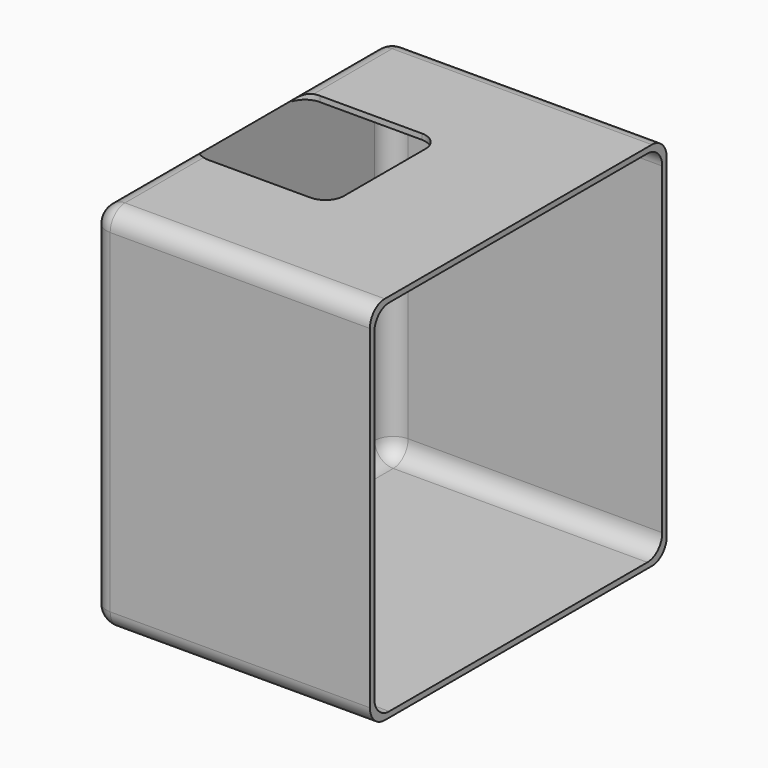
from build123d import *

# Parameters (mm, degrees)
F0_W          = 101.6
F0_H          = 101.6
F0_W_2        = 98.552
F0_H_2        = 98.552
F1_DEPTH      = 76.2
F2_W          = 101.6
F2_H          = 101.6
F3_DEPTH      = 1.524
F4_W          = 38.1
F4_H          = 38.1
F5_DEPTH      = 1.524
F6_R          = 5.08
F7_R          = 5.08
F10_T1_DEPTH  = 93.472
F10_T3_DEPTH  = 88.392
F10_T5_DEPTH  = 74.676
F10_T7_DEPTH  = 69.596
F10_S11_W     = 5.08
F10_S11_H     = 5.08
F10_T12_DEPTH = 5.08
F10_S17_W     = 5.08
F10_S17_H     = 5.08
F10_T18_DEPTH = 5.08
F10_T21_DEPTH = 91.44
F10_T23_DEPTH = 91.44
F10_T26_ANGLE = 90
F10_T28_ANGLE = 90
F10_T30_ANGLE = 90
F10_T32_ANGLE = 90


# Not quite as in the source:
# - a fillet or chamfer that OpenCascade refuses, or shapes differently, is made with other operations: its cross-section is extruded or revolved along the edge and cut away or added
# - a feature of the source that left no trace in its solid (it failed there, or was rolled back) is left out


with BuildPart() as f1:
    # F0 (on Right) → F1 (new body)
    with BuildSketch(Plane.YZ):
        Rectangle(F0_W, F0_H)
        Rectangle(F0_W_2, F0_H_2, mode=Mode.SUBTRACT)
    extrude(amount=F1_DEPTH)

    # F2 (on Right) → F3 (join)
    with BuildSketch(Plane.YZ):
        Rectangle(F2_W, F2_H)
    extrude(amount=F3_DEPTH)

    # F4 (on face) → F5 (cut)
    with BuildSketch(Plane.XY.offset(50.8)):
        with Locations((20.574, 0)):
            Rectangle(F4_W, F4_H)
    extrude(amount=-F5_DEPTH, mode=Mode.SUBTRACT)

    # F6
    f6_edges = [f1.edges().sort_by_distance(p)[0] for p in [
        (39.624, 19.05, 50.038),
        (39.624, -19.05, 50.038),
        (1.524, -19.05, 50.038),
        (1.524, 19.05, 50.038),
    ]]
    fillet(f6_edges, radius=F6_R)

    # F7
    f7_edges = [f1.edges().sort_by_distance(p)[0] for p in [
        (38.1, 50.8, 50.8),
        (38.1, -50.8, 50.8),
        (38.1, -50.8, -50.8),
        (38.1, 50.8, -50.8),
    ]]
    fillet(f7_edges, radius=F7_R)

    # F10: fillet of radius 5.08 on 15 edges, made by hand

    # F10_s2 → F10_t1 (join)
    with BuildSketch(Plane.XY.offset(-44.196)):
        with BuildLine():
            ThreePointArc((1.524, 44.196), (3.0118975516, 47.7881024484), (6.604, 49.276))
            Line((6.604, 49.276), (1.524, 49.276))
            Line((1.524, 49.276), (1.524, 44.196))
        make_face()
        with BuildLine():
            ThreePointArc((1.524, -44.196), (3.0118975516, -47.7881024484), (6.604, -49.276))
            Line((6.604, -49.276), (1.524, -49.276))
            Line((1.524, -49.276), (1.524, -44.196))
        make_face()
    extrude(amount=F10_T1_DEPTH)

    # F10_s4 → F10_t3 (join)
    with BuildSketch(Plane.XZ.offset(-44.196)):
        with BuildLine():
            ThreePointArc((1.524, -44.196), (3.0118975516, -47.7881024484), (6.604, -49.276))
            Line((6.604, -49.276), (1.524, -49.276))
            Line((1.524, -49.276), (1.524, -44.196))
        make_face()
    extrude(amount=F10_T3_DEPTH)

    # F10_s6 → F10_t5 (join)
    with BuildSketch(Plane.YZ.offset(1.524)):
        with BuildLine():
            ThreePointArc((-49.276, 44.196), (-47.7881024484, 47.7881024484), (-44.196, 49.276))
            Line((-44.196, 49.276), (-49.276, 49.276))
            Line((-49.276, 49.276), (-49.276, 44.196))
        make_face()
        with BuildLine():
            ThreePointArc((44.196, 49.276), (47.7881024484, 47.7881024484), (49.276, 44.196))
            Line((49.276, 44.196), (49.276, 49.276))
            Line((49.276, 49.276), (44.196, 49.276))
        make_face()
    extrude(amount=F10_T5_DEPTH)

    # F10_s8 → F10_t7 (join)
    with BuildSketch(Plane.YZ.offset(6.604)):
        with BuildLine():
            ThreePointArc((-49.276, -44.196), (-47.7881024484, -47.7881024484), (-44.196, -49.276))
            Line((-44.196, -49.276), (-49.276, -49.276))
            Line((-49.276, -49.276), (-49.276, -44.196))
        make_face()
        with BuildLine():
            ThreePointArc((49.276, -44.196), (47.7881024484, -47.7881024484), (44.196, -49.276))
            Line((44.196, -49.276), (49.276, -49.276))
            Line((49.276, -49.276), (49.276, -44.196))
        make_face()
    extrude(amount=F10_T7_DEPTH)


with BuildPart() as f10_tool10:
    # F10_s11 → F10_t12 (new body)
    with BuildSketch(Plane.XY.offset(-44.196)):
        with Locations((4.064, 46.736)):
            Rectangle(F10_S11_W, F10_S11_H)
    extrude(amount=-F10_T12_DEPTH)

    # F10_s13 → F10_t14 (revolve, cut)
    with BuildSketch(Plane(origin=(6.604, 44.196, -44.196), x_dir=(0.7071067812, -0.7071067812, 0), z_dir=(0.7071067812, 0.7071067812, 0))):
        with BuildLine():
            ThreePointArc((0, -5.08), (5.08, 0), (0, 5.08))
            Line((0, 5.08), (0, -5.08))
        make_face()
    revolve(axis=Axis((6.604, 44.196, -44.196), (0, 0, -1)), mode=Mode.SUBTRACT)


with BuildPart() as f1_1:
    add(f1.part)

    # F10_t9: union F10_tool10
    add(f10_tool10.part)


with BuildPart() as f10_tool16:
    # F10_s17 → F10_t18 (new body)
    with BuildSketch(Plane.XY.offset(-44.196)):
        with Locations((4.064, -46.736)):
            Rectangle(F10_S17_W, F10_S17_H)
    extrude(amount=-F10_T18_DEPTH)

    # F10_s19 → F10_t20 (revolve, cut)
    with BuildSketch(Plane(origin=(6.604, -44.196, -44.196), x_dir=(0.7071067812, 0.7071067812, 0), z_dir=(-0.7071067812, 0.7071067812, 0))):
        with BuildLine():
            ThreePointArc((0, -5.08), (5.08, 0), (0, 5.08))
            Line((0, 5.08), (0, -5.08))
        make_face()
    revolve(axis=Axis((6.604, -44.196, -44.196), (0, 0, -1)), mode=Mode.SUBTRACT)


with BuildPart() as f1_2:
    add(f1_1.part)

    # F10_t15: union F10_tool16
    add(f10_tool16.part)

    # F10_s22 → F10_t21 (cut)
    with BuildSketch(Plane.XZ.offset(-45.72)):
        with BuildLine():
            ThreePointArc((5.08, 50.8), (1.4878975516, 49.3121024484), (0, 45.72))
            Line((0, 45.72), (0, 50.8))
            Line((0, 50.8), (5.08, 50.8))
        make_face()
        with BuildLine():
            ThreePointArc((5.08, -50.8), (1.4878975516, -49.3121024484), (0, -45.72))
            Line((0, -45.72), (0, -50.8))
            Line((0, -50.8), (5.08, -50.8))
        make_face()
    extrude(amount=F10_T21_DEPTH, mode=Mode.SUBTRACT)

    # F10_s24 → F10_t23 (cut)
    with BuildSketch(Plane.XY.offset(-45.72)):
        with BuildLine():
            ThreePointArc((5.08, 50.8), (1.4878975516, 49.3121024484), (0, 45.72))
            Line((0, 45.72), (0, 50.8))
            Line((0, 50.8), (5.08, 50.8))
        make_face()
        with BuildLine():
            ThreePointArc((5.08, -50.8), (1.4878975516, -49.3121024484), (0, -45.72))
            Line((0, -45.72), (0, -50.8))
            Line((0, -50.8), (5.08, -50.8))
        make_face()
    extrude(amount=F10_T23_DEPTH, mode=Mode.SUBTRACT)

    # F10_s25 → F10_t26 (revolve, cut)
    with BuildSketch(Plane.XY.offset(-45.72)):
        with BuildLine():
            ThreePointArc((5.08, 50.8), (1.4878975516, 49.3121024484), (0, 45.72))
            Line((0, 45.72), (0, 50.8))
            Line((0, 50.8), (5.08, 50.8))
        make_face()
    revolve(axis=Axis((0, 45.72, -45.72), (-1, 0, 0)), revolution_arc=F10_T26_ANGLE, mode=Mode.SUBTRACT)

    # F10_s27 → F10_t28 (revolve, cut)
    with BuildSketch(Plane.XZ.offset(-45.72)):
        with BuildLine():
            ThreePointArc((5.08, 50.8), (1.4878975516, 49.3121024484), (0, 45.72))
            Line((0, 45.72), (0, 50.8))
            Line((0, 50.8), (5.08, 50.8))
        make_face()
    revolve(axis=Axis((0, 45.72, 45.72), (-1, 0, 0)), revolution_arc=F10_T28_ANGLE, mode=Mode.SUBTRACT)

    # F10_s29 → F10_t30 (revolve, cut)
    with BuildSketch(Plane.XY.offset(-45.72)):
        with BuildLine():
            ThreePointArc((5.08, -50.8), (1.4878975516, -49.3121024484), (0, -45.72))
            Line((0, -45.72), (0, -50.8))
            Line((0, -50.8), (5.08, -50.8))
        make_face()
    revolve(axis=Axis((0, -45.72, -45.72), (1, 0, 0)), revolution_arc=F10_T30_ANGLE, mode=Mode.SUBTRACT)

    # F10_s31 → F10_t32 (revolve, cut)
    with BuildSketch(Plane.XZ.offset(45.72)):
        with BuildLine():
            ThreePointArc((5.08, 50.8), (1.4878975516, 49.3121024484), (0, 45.72))
            Line((0, 45.72), (0, 50.8))
            Line((0, 50.8), (5.08, 50.8))
        make_face()
    revolve(axis=Axis((0, -45.72, 45.72), (1, 0, 0)), revolution_arc=F10_T32_ANGLE, mode=Mode.SUBTRACT)


solid = f1_2.part
